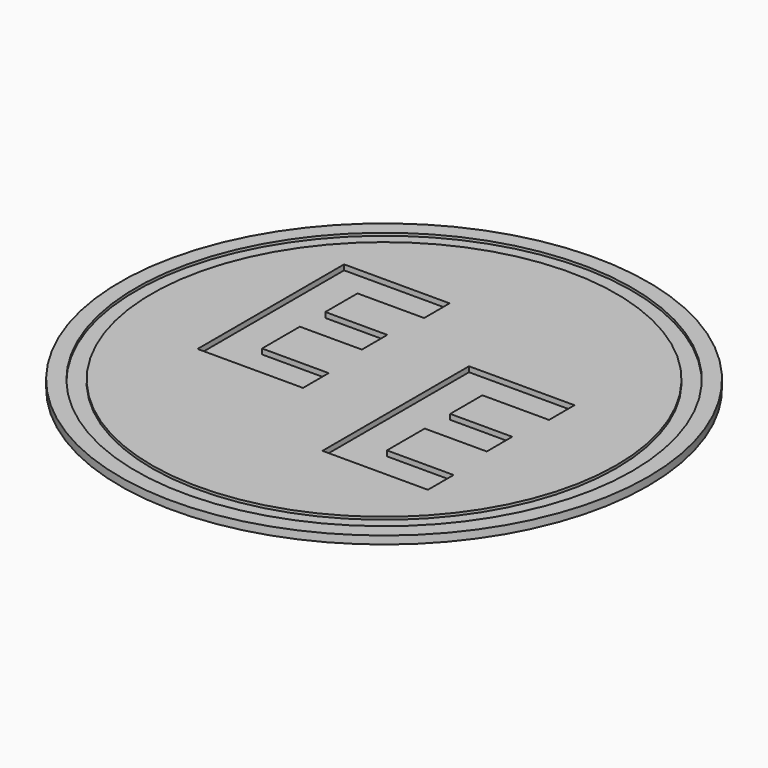
from build123d import *

# Parameters (mm, degrees)
F0_R         = 50
F1_DEPTH     = 1.5
F2_R         = 47
F2_R_2       = 44
F3_DEPTH     = 0.5
F4_TEXT_SIZE = 48.6111111111
F5_DEPTH     = 1
F6_TEXT_SIZE = 48.6111111111
F7_DEPTH     = 1


# Not quite as in the source:
# - Text() gives the source's letters only with a copy of the font that has no kerning and outlines rounded to 1/6400 em; it was checked with that copy


with BuildPart() as f1:
    # F0 (on Top) → F1 (new body)
    with BuildSketch(Plane.XY):
        Circle(F0_R)
    extrude(amount=F1_DEPTH)

    # F2 (on face) → F3 (cut)
    with BuildSketch(Plane.XY.offset(1.5)):
        Circle(F2_R)
        Circle(F2_R_2, mode=Mode.SUBTRACT)
    extrude(amount=-F3_DEPTH, mode=Mode.SUBTRACT)

    # F4 (on face) → F5 (cut)
    with BuildSketch(Plane.XY.offset(1.5)):
        with Locations((-32.0225606839, -9.6026217469)):
            Text('E', F4_TEXT_SIZE, font='Open Sans', font_style=FontStyle.BOLD, text_align=(TextAlign.LEFT, TextAlign.BOTTOM))
    extrude(amount=-F5_DEPTH, mode=Mode.SUBTRACT)

    # F6 (on face) → F7 (cut)
    with BuildSketch(Plane.XY.offset(1.5)):
        with Locations((2.7927289324, -23.5479342469)):
            Text('E', F6_TEXT_SIZE, font='Open Sans', font_style=FontStyle.BOLD, text_align=(TextAlign.LEFT, TextAlign.BOTTOM))
    extrude(amount=-F7_DEPTH, mode=Mode.SUBTRACT)


solid = f1.part
